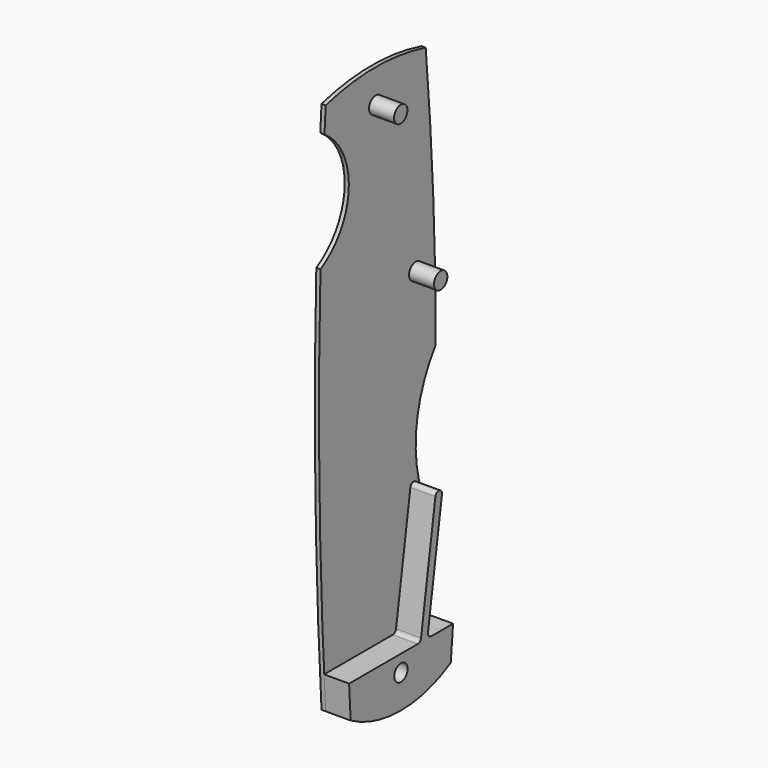
from build123d import *

# Parameters (mm, degrees)
F0_R          = 1.5875
F1_DEPTH      = 0.79375
F2_DEPTH      = 4.7625
F2_DEPTH_BACK = 1.5875
F3_DEPTH      = 4.7625
F4_R          = 0.79374
F7_D          = 3.175
F7_2_D        = 3.175


# Not quite as in the source:
# - a fillet or chamfer is up to 0.001 mm smaller than in the source, because OpenCascade refuses the exact size


with BuildPart() as f1:
    # F0 (on Right) → F1 (new body)
    with BuildSketch(Plane.YZ):
        with BuildLine():
            ThreePointArc((-11.90625, -50.8), (0, -53.975), (11.90625, -50.8))
            ThreePointArc((11.90625, -50.8), (12.8347328861, -39.6958564126), (13.5351884021, -28.575))
            ThreePointArc((13.5351884021, -28.575), (9.5277768783, -14.1720911273), (14.2875, 0))
            ThreePointArc((14.2875, 0), (13.6918608439, 25.4278899614), (11.90625, 50.8))
            ThreePointArc((11.90625, 50.8), (0, 52.3875), (-11.90625, 50.8))
            ThreePointArc((-11.90625, 50.8), (-12.0517066, 48.4189581239), (-12.1901812978, 46.0375))
            ThreePointArc((-12.1901812978, 46.0375), (-6.4020679088, 34.6659483313), (-13.1445991419, 23.8330024471))
            ThreePointArc((-13.1445991419, 23.8330024471), (-13.381777253, -13.4977078204), (-11.90625, -50.8))
        make_face()
        with Locations((0, 46.0375)):
            Circle(F0_R, mode=Mode.SUBTRACT)
        with Locations((9.525, 14.2875)):
            Circle(F0_R, mode=Mode.SUBTRACT)
    extrude(amount=-F1_DEPTH)

    # F7 (through all)
    with Locations(Plane.YZ.offset(4.7625)):
        with Locations((0.0482433617, -47.6255920894)):
            Hole(F7_D / 2)


with BuildPart() as f2:
    # F0 (on Right) → F2 (new body, two sides)
    with BuildSketch(Plane.YZ) as f2_sk:
        with Locations((0, 46.0375)):
            Circle(F0_R)
    extrude(amount=F2_DEPTH)
    extrude(f2_sk.sketch, amount=-F2_DEPTH_BACK)


with BuildPart() as f2b:
    # F0 (on Right) → F2, piece 2 (new body, two sides)
    with BuildSketch(Plane.YZ) as f2_2_sk:
        with Locations((9.525, 14.2875)):
            Circle(F0_R)
    extrude(amount=F2_DEPTH)
    extrude(f2_2_sk.sketch, amount=-F2_DEPTH_BACK)


with BuildPart() as f3:
    # F6 (on face) → F3 (new body)
    with BuildSketch(Plane.YZ):
        with BuildLine():
            Line((4.744096871, -44.45), (-12.2785986466, -44.45))
            ThreePointArc((-12.2785986466, -44.45), (-12.0986301104, -47.6253638923), (-11.90625, -50.8))
            ThreePointArc((-11.90625, -50.8), (0, -53.975), (11.90625, -50.8))
            ThreePointArc((11.90625, -50.8), (12.1950900719, -47.6258202864), (12.4652954557, -44.45))
            Line((12.4652954557, -44.45), (6.35, -44.45))
            Line((6.35, -44.45), (4.744096871, -44.45))
        make_face()
        Polygon((8.3753566937, -20.6707392301), (4.744096871, -44.45), (6.35, -44.45), (9.9446644586, -20.9103835273), align=None)
    extrude(amount=F3_DEPTH)

    # F4 (radius 0.79375 in the source; OpenCascade refuses exactly that, so slightly less here)
    f4_edges = [f3.edges().sort_by_distance(p)[0] for p in [
        (2.38125, 4.744097, -44.45),
        (2.38125, 6.35, -44.45),
        (2.38125, 9.944664, -20.910384),
        (2.38125, 8.375357, -20.670739),
    ]]
    fillet(f4_edges, radius=F4_R)

    # F7#2 (through all)
    with Locations(Plane.YZ.offset(4.7625)):
        with Locations((0.0482433617, -47.6255920894)):
            Hole(F7_2_D / 2)


solid = Compound([f1.part, f2.part, f2b.part, f3.part])
